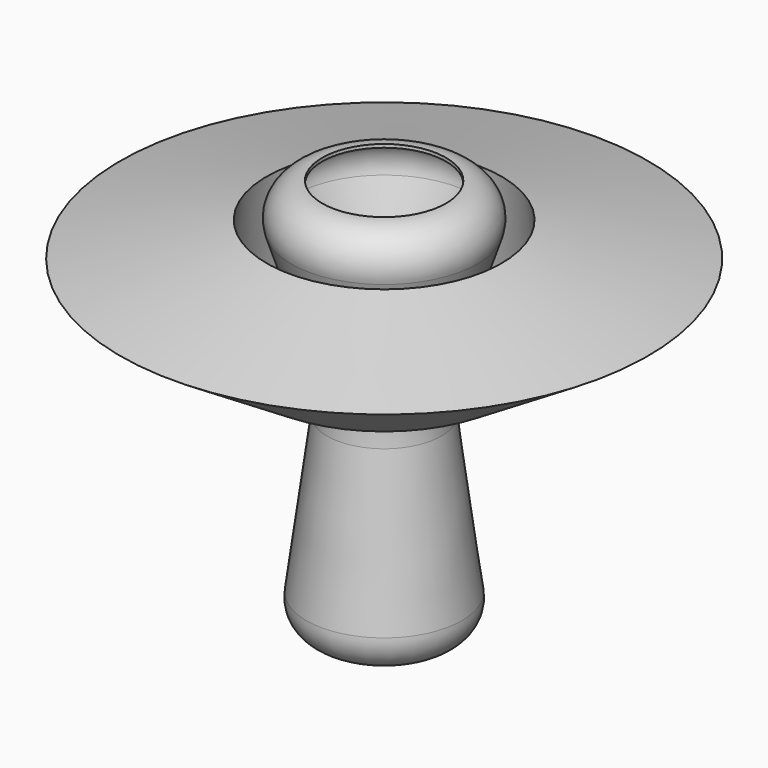
from build123d import *

# Parameters (mm, degrees)
F2_R = 5.08
F3_R = 5.08
F4_T = -0.508


# Not quite as in the source:
# - a shell that OpenCascade refuses in one call is made with other operations: the cavity is built on its own and cut out


with BuildPart() as f1:
    # F0 (on Right) → F1 (revolve)
    with BuildSketch(Plane.YZ):
        with BuildLine():
            Line((0, -32.2118587792), (0, 29.4477399439))
            Line((0, 29.4477399439), (-2.8095957153, 29.4477399439))
            Line((-2.8095957153, 29.4477399439), (-16.535570845, 29.4477399439))
            Line((-16.535570845, 29.4477399439), (-9.8354473889, 8.7265070489))
            ThreePointArc((-9.8354473889, 8.7265070489), (-8.7077256174, 3.2112280279), (-8.8225213679, -2.4169938057))
            Line((-8.8225213679, -2.4169938057), (-12.7613620927, -32.2118587792))
            Line((-12.7613620927, -32.2118587792), (0, -32.2118587792))
        make_face()
    revolve(axis=Axis((0, 0, -1.3820594177), (0, 0, -1)))

    # F2
    f2_edges = [f1.edges().sort_by_distance(p)[0] for p in [
        (0, 16.535571, 29.44774),
    ]]
    fillet(f2_edges, radius=F2_R)

    # F3
    f3_edges = [f1.edges().sort_by_distance(p)[0] for p in [
        (0, 12.761362, -32.211859),
    ]]
    fillet(f3_edges, radius=F3_R)

    # F4: a shell. OpenCascade refuses it in one call, so the cavity is built on its own and cut out:
    # the body offset inwards by the wall thickness, plus a prism from it out through each open face.
    f4_core = offset(f1.part, amount=F4_T, mode=Mode.PRIVATE)
    f4_exits = [f4_core.faces().sort_by_distance(p)[0] for p in [
        (0, 0, 28.93974),
        (0, 0, -31.703859),
    ]]
    add(f4_core, mode=Mode.SUBTRACT)
    extrude(f4_exits, amount=-F4_T, mode=Mode.SUBTRACT)


with BuildPart() as f1b:
    # F0 (on Right) → F1, piece 2 (revolve)
    with BuildSketch(Plane.YZ):
        Polygon((40.7538414001, 18.8644435257), (18.1377814998, 24.1019894291), (19.5579826832, 5.523710046), align=None)
    revolve(axis=Axis((0, 0, -1.3820594177), (0, 0, -1)))


solid = Compound([f1.part, f1b.part])
